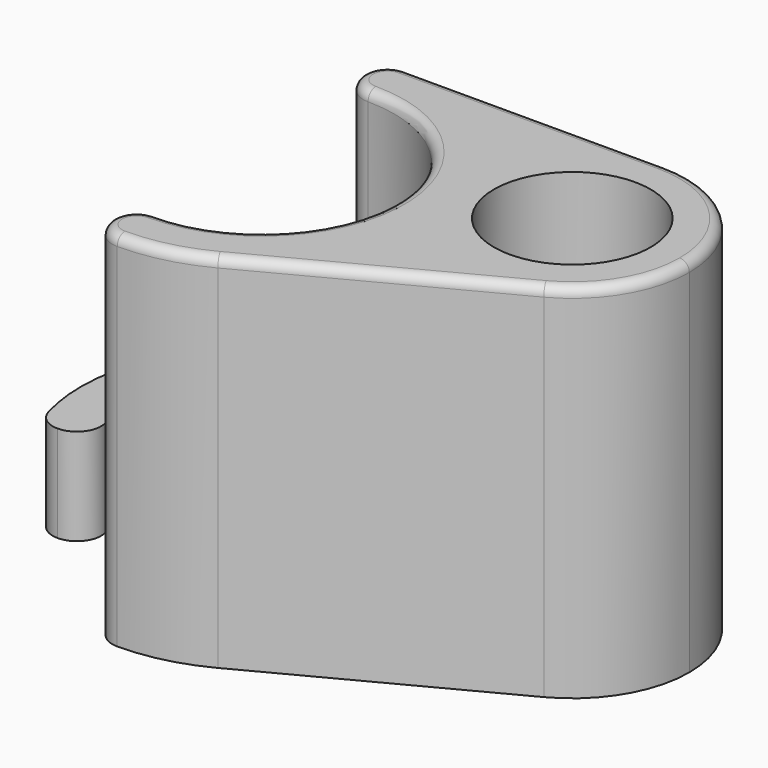
from build123d import *

# Parameters (mm, degrees)
F1_DEPTH = 4
F2_R     = 1
F3_DEPTH = 11
F5_DEPTH = 15
F6_R     = 0.99999
F7_R     = 0.4


# Not quite as in the source:
# - a fillet or chamfer that OpenCascade refuses, or shapes differently, is made with other operations: its cross-section is extruded or revolved along the edge and cut away or added
# - a fillet or chamfer is up to 0.001 mm smaller than in the source, because OpenCascade refuses the exact size
# - a feature names something its author has since deleted; it is built from what else it names


with BuildPart() as f1:
    # F0 (on Top) → F1 (new body)
    with BuildSketch(Plane.XY):
        with BuildLine():
            ThreePointArc((-4.75, -2.7726341266), (-1.4361406616, 5.3091901454), (5.5, 0))
            ThreePointArc((5.5, 0), (5.3091901454, -1.4361406616), (4.75, -2.7726341266))
            Line((4.75, -2.7726341266), (6.9686799324, -2.7726341266))
            ThreePointArc((6.9686799324, -2.7726341266), (7.3659724237, -1.4115418001), (7.5, 0))
            ThreePointArc((7.5, 0), (5.3033008589, 5.3033008589), (0, 7.5))
            ThreePointArc((0, 7.5), (-5.3033008589, 5.3033008589), (-7.5, 0))
            ThreePointArc((-7.5, 0), (-7.3659724237, -1.4115418001), (-6.9686799324, -2.7726341266))
            Line((-6.9686799324, -2.7726341266), (-4.75, -2.7726341266))
        make_face()
        with BuildLine():
            ThreePointArc((0, 7.5), (5.3033008589, 5.3033008589), (7.5, 0))
            Line((7.5, 0), (7.5, 7.5))
            Line((7.5, 7.5), (0, 7.5))
        make_face()
    extrude(amount=F1_DEPTH)

    # F2 (on face) → F3 (join)
    with BuildSketch(Plane.XY.offset(4)):
        with Locations((0, 6.5)):
            Circle(F2_R)
        with BuildLine():
            ThreePointArc((0, 7.5), (0.7071067812, 7.2071067812), (1, 6.5))
            ThreePointArc((1, 6.5), (0.7071067812, 5.7928932188), (0, 5.5))
            ThreePointArc((0, 5.5), (4.769669155, 2.7386595538), (4.75, -2.7726341266))
            Line((4.75, -2.7726341266), (6.9686799324, -2.7726341266))
            ThreePointArc((6.9686799324, -2.7726341266), (7.3659724237, -1.4115418001), (7.5, 0))
            Line((7.5, 0), (7.5, 7.5))
            Line((7.5, 7.5), (0, 7.5))
        make_face()
    extrude(amount=F3_DEPTH)

    # F4 (on face) → F5 (join, through all)
    with BuildSketch(Plane.XY.offset(15)):
        with BuildLine():
            Line((7.5, 6.25), (7.5, 2.65))
            Line((7.5, 2.65), (7.5, 0))
            ThreePointArc((7.5, 0), (7.4864300086, -0.4509608915), (7.4457691398, -0.9002899069))
            ThreePointArc((7.4457691398, -0.9002899069), (10.1065360675, -2.1571253539), (13.0041807725, -1.6443182282))
            ThreePointArc((13.0041807725, -1.6443182282), (14.900619035, 0.1410437177), (15.6, 2.65))
            ThreePointArc((15.6, 2.65), (14.1794678888, 6.0794678888), (10.75, 7.5))
            ThreePointArc((10.75, 7.5), (9.0089514654, 7.1767261901), (7.5, 6.25))
        make_face()
        with BuildLine():
            ThreePointArc((7.5, 2.65), (10.75, 5.9), (14, 2.65))
            ThreePointArc((14, 2.65), (10.75, -0.6), (7.5, 2.65))
        make_face(mode=Mode.SUBTRACT)
        with BuildLine():
            Line((7.5, 0), (7.5, 2.65))
            Line((7.5, 2.65), (7.5, 6.25))
            ThreePointArc((7.5, 6.25), (6.712321746, 5.3369414428), (6.1742445242, 4.2577816473))
            ThreePointArc((6.1742445242, 4.2577816473), (7.1608949836, 2.2297046967), (7.5, 0))
        make_face()
        with BuildLine():
            ThreePointArc((7.4457691398, -0.9002899069), (7.4864300086, -0.4509608915), (7.5, 0))
            ThreePointArc((7.5, 0), (7.1608949836, 2.2297046967), (6.1742445242, 4.2577816473))
            ThreePointArc((6.1742445242, 4.2577816473), (6.0409691333, 1.4891691352), (7.4457691398, -0.9002899069))
        make_face()
        with BuildLine():
            Line((7.5, 7.5), (7.5, 6.25))
            ThreePointArc((7.5, 6.25), (9.0089514654, 7.1767261901), (10.75, 7.5))
            Line((10.75, 7.5), (7.5, 7.5))
        make_face()
        with BuildLine():
            ThreePointArc((13.0041807725, -1.6443182282), (10.1065360675, -2.1571253539), (7.4457691398, -0.9002899069))
            ThreePointArc((7.4457691398, -0.9002899069), (7.2677715796, -1.8518899176), (6.9686799324, -2.7726341266))
            ThreePointArc((6.9686799324, -2.7726341266), (5.5735770486, -5.0184897015), (3.4858465555, -6.640698291))
            Line((3.4858465555, -6.640698291), (13.0041807725, -1.6443182282))
        make_face()
        with BuildLine():
            ThreePointArc((3.4858465555, -6.640698291), (5.5735770486, -5.0184897015), (6.9686799324, -2.7726341266))
            Line((6.9686799324, -2.7726341266), (4.75, -2.7726341266))
            ThreePointArc((4.75, -2.7726341266), (2.7386595462, -4.7696691594), (-1.76e-08, -5.5))
            ThreePointArc((-1.76e-08, -5.5), (0.707106775, -5.7928932126), (1, -6.5))
            ThreePointArc((1, -6.5), (0.7071067812, -7.2071067812), (0, -7.5))
            ThreePointArc((0, -7.5), (1.7950992755, -7.2820064949), (3.4858465555, -6.640698291))
        make_face()
        with BuildLine():
            ThreePointArc((-1.76e-08, -5.5), (-1, -6.5000000088), (0, -7.5))
            ThreePointArc((0, -7.5), (0.7071067812, -7.2071067812), (1, -6.5))
            ThreePointArc((1, -6.5), (0.707106775, -5.7928932126), (-1.76e-08, -5.5))
        make_face()
    extrude(amount=-F5_DEPTH)

    # F6 (radius 1 in the source; OpenCascade refuses exactly that, so slightly less here)
    f6_edges = [f1.edges().sort_by_distance(p)[0] for p in [
        (-6.96868, -2.772634, 2),
        (-4.75, -2.772634, 2),
    ]]
    fillet(f6_edges, radius=F6_R)

    # F7
    f7_edges = [f1.edges().sort_by_distance(p)[0] for p in [
        (8.245014, -4.142508, 15),
        (3.75, 7.5, 15),
        (4.769669, 2.73866, 15),
        (-1, 6.5, 15),
        (9.125, 7.5, 15),
        (15.459031, 3.810831, 15),
        (1.795099, -7.282006, 15),
        (-1, -6.5, 15),
        (2.73866, -4.769669, 15),
    ]]
    fillet(f7_edges, radius=F7_R)

    # F8: chamfer of 1 on 1 edges, made by hand

    # F8_s1 → F8_t2 (revolve, cut)
    with BuildSketch(Plane.XZ.offset(-2.65)):
        Polygon((6.5, 0), (7.5, 1), (7.5, 0), align=None)
    revolve(axis=Axis((10.75, 2.65, 0), (0, 0, -1)), mode=Mode.SUBTRACT)

    # F9: fillet of radius 20 on 1 edges, made by hand

    # F9_s1 → F9_t2 (revolve, cut)
    with BuildSketch(Plane.XZ.offset(-2.65)):
        with BuildLine():
            ThreePointArc((7.5, 6.2449979984), (7.2484176581, 3.0827203382), (6.5, 0))
            Line((6.5, 0), (7.5, 1))
            Line((7.5, 1), (7.5, 6.2449979984))
        make_face()
    revolve(axis=Axis((10.75, 2.65, 1), (0, 0, -1)), mode=Mode.SUBTRACT)


solid = f1.part
